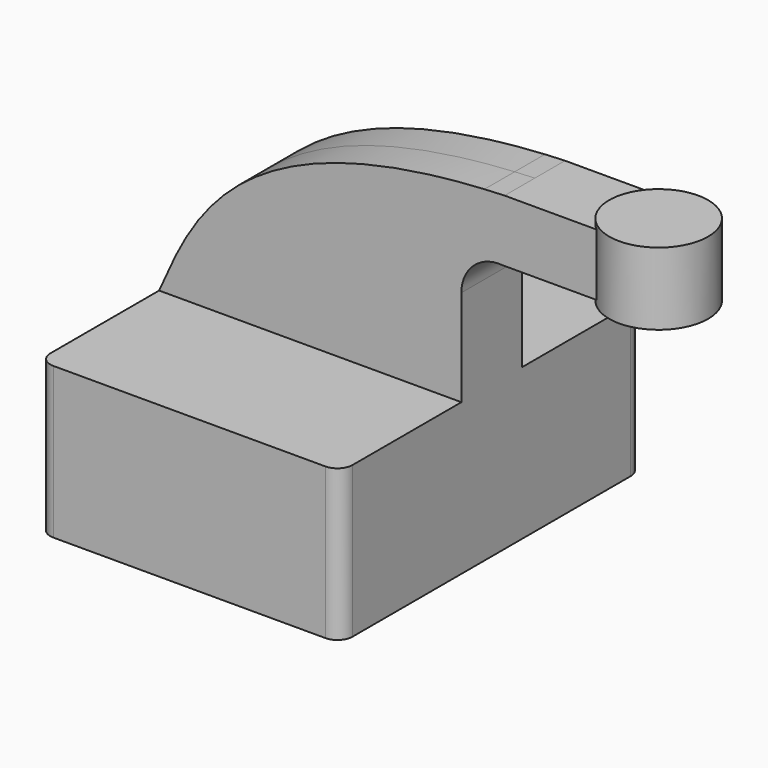
from build123d import *

# Parameters (mm, degrees)
F1_DEPTH = 63.5
F0_W     = 17.5679588894
F0_H     = 20.8251091272
F2_DEPTH = 12.7
F4_R     = 5.08
F5_R     = 5.08


with BuildPart() as f1:
    # F0 (on Front) → F1 (new body, symmetric)
    with BuildSketch(Plane.XZ):
        Polygon((-50.8, 25.4), (-50.8, -25.4), (50.8, -25.4), (50.8, 25.4), (29.9748908728, 25.4), align=None)
    extrude(amount=F1_DEPTH, both=True)

    # F0 (on Front) → F2 (join, symmetric)
    with BuildSketch(Plane.XZ):
        with BuildLine():
            add(Edge.make_bspline(
                [(-50.8, 25.4), (-40.0576822889, 49.6242242179), (-26.1354784037, 86.069146105), (58.5620329332, 90.9465027441)],
                knots=[0, 0, 0, 0, 130.1130965779, 130.1130965779, 130.1130965779, 130.1130965779], degree=3))
            Line((-50.8, 25.4), (29.9748908728, 25.4))
            Line((29.9748908728, 25.4), (29.9748908728, 57.7870482366))
            ThreePointArc((29.9748908728, 57.7870482366), (38.1082806139, 79.6775376922), (58.5620329332, 90.9465027441))
        make_face()
        with BuildLine():
            Line((29.9748908728, 25.4), (50.8, 25.4))
            Line((50.8, 25.4), (50.8, 57.7870482366))
            ThreePointArc((50.8, 57.7870482366), (54.9254885829, 67.1554928224), (64.6216935366, 70.4374159629))
            Line((64.6216935366, 70.4374159629), (89.3876225336, 70.4374159629))
            Line((89.3876225336, 70.4374159629), (89.3876225336, 91.2625250901))
            Line((89.3876225336, 91.2625250901), (65.3235655796, 91.2625250901))
            add(Edge.make_bspline(
                [(58.5620329332, 90.9465027441), (60.7674907461, 91.0735053459), (63.0209371473, 91.1791038317), (65.3235655796, 91.2625250901)],
                knots=[130.1130965779, 130.1130965779, 130.1130965779, 130.1130965779, 133.5011411718, 133.5011411718, 133.5011411718, 133.5011411718], degree=3))
            ThreePointArc((58.5620329332, 90.9465027441), (38.1082806139, 79.6775376922), (29.9748908728, 57.7870482366))
            Line((29.9748908728, 57.7870482366), (29.9748908728, 25.4))
        make_face()
        with Locations((98.1716019783, 80.8499705265)):
            Rectangle(F0_W, F0_H)
    extrude(amount=F2_DEPTH, both=True)

    # F0 (on Front) → F3 (revolve)
    with BuildSketch(Plane.XZ):
        Polygon((106.955581423, 92.8989347667), (106.955581423, 91.2625250901), (106.955581423, 70.4374159629), (106.955581423, 68.5675365603), (123.5830926897, 68.5675365603), (123.5830926897, 92.8989347667), align=None)
    revolve(axis=Axis((106.955581423, 0, 80.7332356635), (0, 0, -1)))

    # F4
    f4_edges = [f1.edges().sort_by_distance(p)[0] for p in [
        (50.8, -63.5, 0),
        (-50.8, -63.5, 0),
        (50.8, 63.5, 0),
    ]]
    fillet(f4_edges, radius=F4_R)

    # F5
    f5_edges = [f1.edges().sort_by_distance(p)[0] for p in [
        (-50.8, 63.5, 0),
    ]]
    fillet(f5_edges, radius=F5_R)


solid = f1.part
